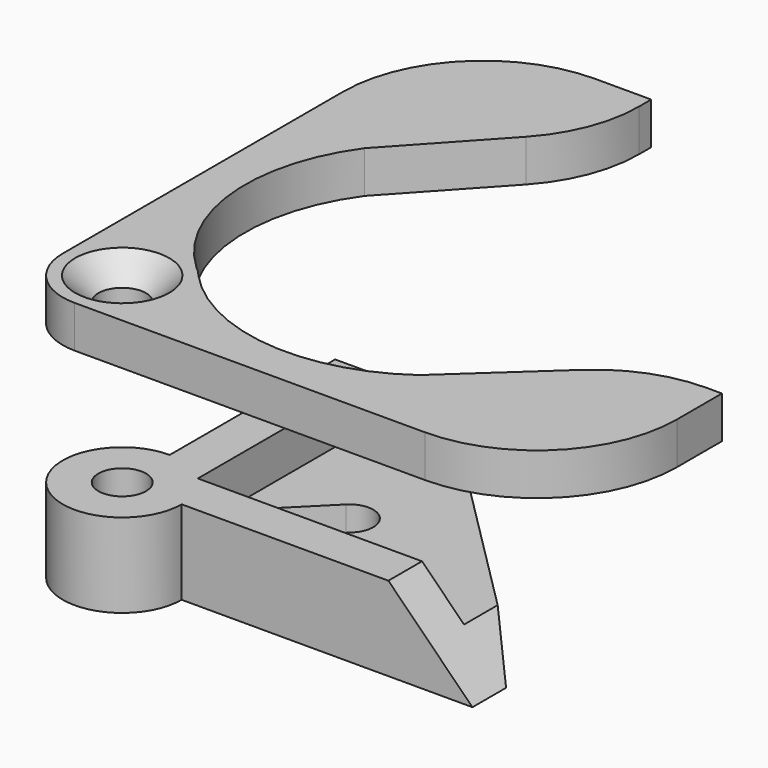
from build123d import *

# Parameters (mm, degrees)
F1_DEPTH         = 3
F2_DEPTH         = 3
F5_DEPTH         = 3
F7_D             = 3.4
F7_DEPTH         = 50
F7_CSINK_D       = 6.72
F7_CSINK_ANGLE   = 90
F7_TIP           = 1.0214630523
F7_2_D           = 3.4
F7_2_DEPTH       = 50
F7_2_CSINK_D     = 6.72
F7_2_CSINK_ANGLE = 90
F7_2_TIP         = 1.0214630523
F9_DEPTH         = 2
F10_R            = 10
F11_T1_DEPTH     = 33.8601958556
F11_T3_DEPTH     = 33.8601958556


# Not quite as in the source:
# - a fillet or chamfer that OpenCascade refuses, or shapes differently, is made with other operations: its cross-section is extruded or revolved along the edge and cut away or added
# - a feature names something its author has since deleted; it is built from what else it names


with BuildPart() as f1:
    # F0 (on Top) → F1 (new body)
    with BuildSketch(Plane.XY):
        with BuildLine():
            ThreePointArc((-12.5, -8.2573593129), (-10.8764116996, -8.5803111054), (-9.5, -9.5))
            Line((-9.5, -9.5), (-9.5, 12.5))
            Line((-9.5, 12.5), (-12.5, 12.5))
            Line((-12.5, 12.5), (-12.5, -8.2573593129))
        make_face()
        with BuildLine():
            Line((-8.2573593129, -12.5), (12.5, -12.5))
            Line((12.5, -12.5), (12.5, -9.5))
            Line((12.5, -9.5), (-9.5, -9.5))
            ThreePointArc((-9.5, -9.5), (-8.5803111054, -10.8764116996), (-8.2573593129, -12.5))
        make_face()
        with BuildLine():
            Line((-12.5, -12.5), (-8.2573593129, -12.5))
            ThreePointArc((-8.2573593129, -12.5), (-8.5803111054, -10.8764116996), (-9.5, -9.5))
            ThreePointArc((-9.5, -9.5), (-10.8764116996, -8.5803111054), (-12.5, -8.2573593129))
            Line((-12.5, -8.2573593129), (-12.5, -12.5))
        make_face()
        with BuildLine():
            ThreePointArc((-12.5, -8.2573593129), (-15.5, -15.5), (-8.2573593129, -12.5))
            Line((-8.2573593129, -12.5), (-12.5, -12.5))
            Line((-12.5, -12.5), (-12.5, -8.2573593129))
        make_face()
        Polygon((-9.5, -9.5), (12.5, -9.5), (-9.5, 12.5), align=None)
        with BuildLine():
            Line((-2.2875108319, -4.6916738879), (-5.1159379566, -7.5201010127))
            ThreePointArc((-5.1159379566, -7.5201010127), (-7.5201010127, -7.5201010127), (-7.5201010127, -5.1159379566))
            Line((-7.5201010127, -5.1159379566), (-4.6916738879, -2.2875108319))
            ThreePointArc((-4.6916738879, -2.2875108319), (-2.2875108319, -2.2875108319), (-2.2875108319, -4.6916738879))
        make_face(mode=Mode.SUBTRACT)
    extrude(amount=-F1_DEPTH)

    # F0 (on Top) → F2 (join)
    with BuildSketch(Plane.XY):
        with BuildLine():
            ThreePointArc((-12.5, -8.2573593129), (-15.5, -15.5), (-8.2573593129, -12.5))
            Line((-8.2573593129, -12.5), (-12.5, -12.5))
            Line((-12.5, -12.5), (-12.5, -8.2573593129))
        make_face()
        with BuildLine():
            Line((-12.5, -12.5), (-8.2573593129, -12.5))
            ThreePointArc((-8.2573593129, -12.5), (-8.5803111054, -10.8764116996), (-9.5, -9.5))
            ThreePointArc((-9.5, -9.5), (-10.8764116996, -8.5803111054), (-12.5, -8.2573593129))
            Line((-12.5, -8.2573593129), (-12.5, -12.5))
        make_face()
        with BuildLine():
            ThreePointArc((-12.5, -8.2573593129), (-10.8764116996, -8.5803111054), (-9.5, -9.5))
            Line((-9.5, -9.5), (-9.5, 12.5))
            Line((-9.5, 12.5), (-12.5, 12.5))
            Line((-12.5, 12.5), (-12.5, -8.2573593129))
        make_face()
        with BuildLine():
            Line((-8.2573593129, -12.5), (12.5, -12.5))
            Line((12.5, -12.5), (12.5, -9.5))
            Line((12.5, -9.5), (-9.5, -9.5))
            ThreePointArc((-9.5, -9.5), (-8.5803111054, -10.8764116996), (-8.2573593129, -12.5))
        make_face()
    extrude(amount=F2_DEPTH)

    # F7
    with Locations(Plane.XY.offset(16)):
        with Locations((-12.5, -12.5)):
            CounterSinkHole(F7_D / 2, F7_CSINK_D / 2, depth=F7_DEPTH, counter_sink_angle=F7_CSINK_ANGLE)
            with Locations((0, 0, -(F7_DEPTH + F7_TIP / 2))):  # 118° drill point
                Cone(0, F7_D / 2, F7_TIP, mode=Mode.SUBTRACT)

    # F8 (on face) → F9 (cut)
    with BuildSketch(Plane(origin=(0, 0, -3), x_dir=(1, 0, 0), z_dir=(0, 0, -1))):
        Polygon((-13.3666896231, 15.7345297078), (-15.7345297078, 13.3666896231), (-14.8678400847, 10.1321599153), (-11.6333103769, 9.2654702922), (-9.2654702922, 11.6333103769), (-10.1321599153, 14.8678400847), align=None)
    extrude(amount=-F9_DEPTH, mode=Mode.SUBTRACT)

    # F11: chamfer of 6 on 2 edges, made by hand

    # F11_s2 → F11_t1 (cut)
    with BuildSketch(Plane.XZ.offset(-5.9300979278)):
        Polygon((6.5, 3), (12.5, -3), (12.5, 3), align=None)
    extrude(amount=F11_T1_DEPTH, mode=Mode.SUBTRACT)

    # F11_s4 → F11_t3 (cut)
    with BuildSketch(Plane.YZ.offset(-27.9300979278)):
        Polygon((12.5, -3), (6.5, 3), (12.5, 3), align=None)
    extrude(amount=F11_T3_DEPTH, mode=Mode.SUBTRACT)


with BuildPart() as f5:
    # F4 (on offset) → F5 (new body)
    with BuildSketch(Plane.XY.offset(13)):
        with BuildLine():
            ThreePointArc((-9.8464677493, -9.1895972156), (-14.3360305156, -8.6752134771), (-16.7426406871, -12.5))
            ThreePointArc((-16.7426406871, -12.5), (-15.5, -15.5), (-12.5, -16.7426406871))
            ThreePointArc((-12.5, -16.7426406871), (-9.5, -15.5), (-8.2573593129, -12.5))
            ThreePointArc((-8.2573593129, -12.5), (-8.497197885, -11.0937371412), (-9.1895972156, -9.8464677493))
            ThreePointArc((-9.1895972156, -9.8464677493), (-9.3463484327, -9.6746223732), (-9.5, -9.5))
            ThreePointArc((-9.5, -9.5), (-9.6746223732, -9.3463484327), (-9.8464677493, -9.1895972156))
        make_face()
        with BuildLine():
            Line((-16.7426406871, 22.5), (-16.7426406871, -12.5))
            ThreePointArc((-16.7426406871, -12.5), (-14.3360305156, -8.6752134771), (-9.8464677493, -9.1895972156))
            ThreePointArc((-9.8464677493, -9.1895972156), (-13.936348556, -0.9487103143), (-11.5473889556, 7.935670022))
            Line((-11.5473889556, 7.935670022), (-2.7426406871, 17.5))
            Line((-2.7426406871, 17.5), (-2.7426406871, 22.5))
            Line((-2.7426406871, 22.5), (-16.7426406871, 22.5))
        make_face()
        with BuildLine():
            ThreePointArc((-8.2573593129, -12.5), (-9.5, -15.5), (-12.5, -16.7426406871))
            Line((-12.5, -16.7426406871), (22.5, -16.7426406871))
            Line((22.5, -16.7426406871), (22.5, -2.7426406871))
            Line((22.5, -2.7426406871), (17.5, -2.7426406871))
            Line((17.5, -2.7426406871), (7.935670022, -11.5473889556))
            ThreePointArc((7.935670022, -11.5473889556), (-0.9487103143, -13.936348556), (-9.1895972156, -9.8464677493))
            ThreePointArc((-9.1895972156, -9.8464677493), (-8.497197885, -11.0937371412), (-8.2573593129, -12.5))
        make_face()
        with BuildLine():
            ThreePointArc((-9.5, -9.5), (-9.6689764749, -9.3400465509), (-9.8464677493, -9.1895972156))
            ThreePointArc((-9.8464677493, -9.1895972156), (-9.6746223732, -9.3463484327), (-9.5, -9.5))
        make_face()
        with BuildLine():
            ThreePointArc((-9.1895972156, -9.8464677493), (-9.3400465509, -9.6689764749), (-9.5, -9.5))
            ThreePointArc((-9.5, -9.5), (-9.3463484327, -9.6746223732), (-9.1895972156, -9.8464677493))
        make_face()
    extrude(amount=F5_DEPTH)

    # F7#2
    with Locations(Plane.XY.offset(16)):
        with Locations((-12.5, -12.5)):
            CounterSinkHole(F7_2_D / 2, F7_2_CSINK_D / 2, depth=F7_2_DEPTH, counter_sink_angle=F7_2_CSINK_ANGLE)
            with Locations((0, 0, -(F7_2_DEPTH + F7_2_TIP / 2))):  # 118° drill point
                Cone(0, F7_2_D / 2, F7_2_TIP, mode=Mode.SUBTRACT)

    # F10
    f10_edges = [f5.edges().sort_by_distance(p)[0] for p in [
        (-16.742641, 22.5, 14.5),
        (22.5, -16.742641, 14.5),
        (-2.742641, 17.5, 14.5),
        (17.5, -2.742641, 14.5),
    ]]
    fillet(f10_edges, radius=F10_R)


solid = Compound([f1.part, f5.part])
